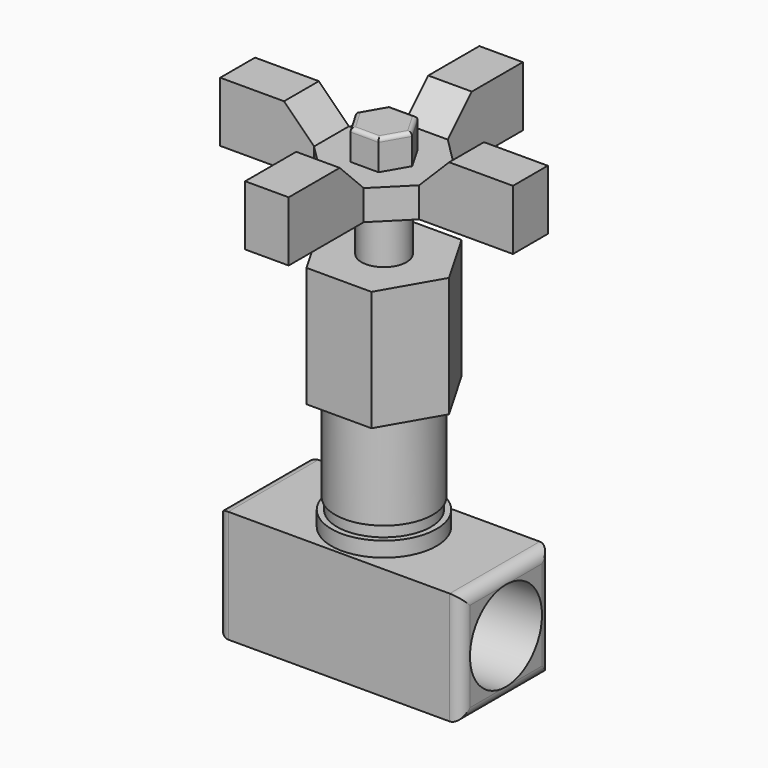
from build123d import *

# Parameters (mm, degrees)
F0_W      = 65
F0_H      = 30
F1_DEPTH  = 30
F2_R      = 12
F3_DEPTH  = 65
F4_R      = 14
F5_DEPTH  = 4
F6_R      = 12.5
F7_DEPTH  = 3
F8_R      = 13
F8_R_2    = 12.5
F9_DEPTH  = 25
F10_R     = 13
F11_DEPTH = 32
F12_R     = 6
F13_DEPTH = 15
F14_R     = 6
F15_DEPTH = 8
F16_DEPTH = 25
F17_DEPTH = 25
F18_DEPTH = 25
F19_DEPTH = 25
F20_W     = 11.5979797464
F20_H     = 25
F20_W_2   = 25
F20_H_2   = 11.5979797464
F21_DEPTH = 8
F22_SIZE  = 7.99999
F23_R     = 2.99999
F24_R     = 2.99999
F26_DEPTH = 8
F27_R     = 1


# Not quite as in the source:
# - a fillet or chamfer is up to 0.001 mm smaller than in the source, because OpenCascade refuses the exact size


with BuildPart() as f1:
    # F0 (on Top) → F1 (new body)
    with BuildSketch(Plane.XY):
        Rectangle(F0_W, F0_H)
    extrude(amount=F1_DEPTH)

    # F2 (on face) → F3 (cut)
    with BuildSketch(Plane.YZ.offset(32.5)):
        with Locations((0, 15)):
            Circle(F2_R)
    extrude(amount=-F3_DEPTH, mode=Mode.SUBTRACT)

    # F4 (on face) → F5 (join)
    with BuildSketch(Plane.XY.offset(30)):
        Circle(F4_R)
    extrude(amount=F5_DEPTH)

    # F6 (on face) → F7 (join)
    with BuildSketch(Plane.XY.offset(34)):
        Circle(F6_R)
    extrude(amount=F7_DEPTH)

    # F8 (on face) → F9 (join)
    with BuildSketch(Plane.XY.offset(37)):
        Circle(F8_R)
        Circle(F8_R_2, mode=Mode.SUBTRACT)
        Circle(F8_R_2)
    extrude(amount=F9_DEPTH)

    # F10 (on face) → F11 (join)
    with BuildSketch(Plane.XY.offset(62)):
        Polygon((17.3205080757, 0), (8.6602540378, 15), (-8.6602540378, 15), (-17.3205080757, 0), (-8.6602540378, -15), (8.6602540378, -15), align=None)
        Circle(F10_R, mode=Mode.SUBTRACT)
        Circle(F10_R)
    extrude(amount=F11_DEPTH)

    # F12 (on face) → F13 (join)
    with BuildSketch(Plane.XY.offset(94)):
        Circle(F12_R)
    extrude(amount=F13_DEPTH)

    # F14 (on face) → F15 (join)
    with BuildSketch(Plane.XY.offset(109)):
        Polygon((5.7989898732, -14), (14, -5.7989898732), (14, 5.7989898732), (5.7989898732, 14), (-5.7989898732, 14), (-14, 5.7989898732), (-14, -5.7989898732), (-5.7989898732, -14), align=None)
        Circle(F14_R, mode=Mode.SUBTRACT)
        Circle(F14_R)
    extrude(amount=F15_DEPTH)

    # F16 (add): a face of the model
    f16_faces = [f1.faces().sort_by_distance(p)[0] for p in [
        (14, 0, 113),
    ]]
    extrude(f16_faces, amount=F16_DEPTH)

    # F17 (add): a face of the model
    f17_faces = [f1.faces().sort_by_distance(p)[0] for p in [
        (0, -14, 113),
    ]]
    extrude(f17_faces, amount=F17_DEPTH)

    # F18 (add): a face of the model
    f18_faces = [f1.faces().sort_by_distance(p)[0] for p in [
        (-14, 0, 113),
    ]]
    extrude(f18_faces, amount=F18_DEPTH)

    # F19 (add): a face of the model
    f19_faces = [f1.faces().sort_by_distance(p)[0] for p in [
        (0, 14, 113),
    ]]
    extrude(f19_faces, amount=F19_DEPTH)

    # F20 (on face) → F21 (join)
    with BuildSketch(Plane.XY.offset(117)):
        with Locations((0, 26.5)):
            Rectangle(F20_W, F20_H)
        with Locations((-26.5, 0)):
            Rectangle(F20_W_2, F20_H_2)
        with Locations((0, -26.5)):
            Rectangle(F20_W, F20_H)
        with Locations((26.5, 0)):
            Rectangle(F20_W_2, F20_H_2)
    extrude(amount=F21_DEPTH)

    # F22 (size 8 in the source; OpenCascade refuses exactly that, so slightly less here)
    f22_edges = [f1.edges().sort_by_distance(p)[0] for p in [
        (-14, 0, 125),
        (0, -14, 125),
        (14, 0, 125),
        (0, 14, 125),
    ]]
    chamfer(f22_edges, length=F22_SIZE)

    # F23 (radius 3 in the source; OpenCascade refuses exactly that, so slightly less here)
    f23_edges = [f1.edges().sort_by_distance(p)[0] for p in [
        (32.5, -15, 15),
        (32.5, 0, 30),
        (32.5, 15, 15),
        (32.5, 0, 0),
    ]]
    fillet(f23_edges, radius=F23_R)

    # F24 (radius 3 in the source; OpenCascade refuses exactly that, so slightly less here)
    f24_edges = [f1.edges().sort_by_distance(p)[0] for p in [
        (-32.5, 0, 30),
        (-32.5, 15, 15),
        (-32.5, -15, 15),
        (-32.5, 0, 0),
    ]]
    fillet(f24_edges, radius=F24_R)

    # F25 (on face) → F26 (join)
    with BuildSketch(Plane.XY.offset(117)):
        Polygon((7.5055534995, 0), (3.7527767497, 6.5), (-3.7527767497, 6.5), (-7.5055534995, 0), (-3.7527767497, -6.5), (3.7527767497, -6.5), align=None)
    extrude(amount=F26_DEPTH)

    # F27
    f27_edges = [f1.edges().sort_by_distance(p)[0] for p in [
        (0, -6.5, 125),
        (-5.629165, -3.25, 125),
        (-5.629165, 3.25, 125),
        (0, 6.5, 125),
        (5.629165, 3.25, 125),
        (5.629165, -3.25, 125),
    ]]
    fillet(f27_edges, radius=F27_R)


solid = f1.part
